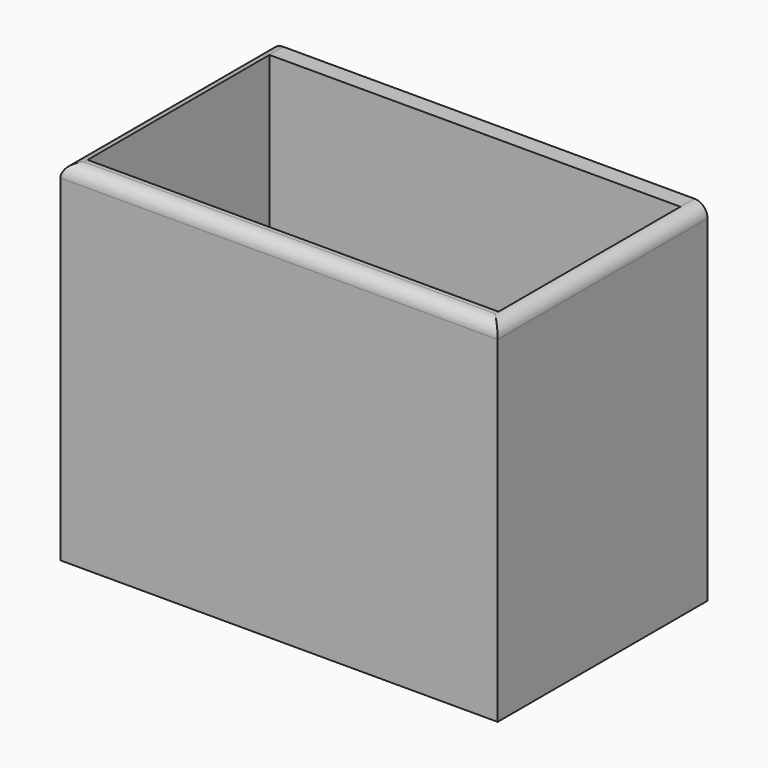
from build123d import *

# Parameters (mm, degrees)
F0_W     = 127
F0_H     = 76.2
F0_W_2   = 119.38
F0_H_2   = 66.04
F1_DEPTH = 101.6
F2_W     = 12.954
F2_H     = 17.78
F3_DEPTH = 5.08
F4_W     = 119.38
F4_H     = 66.04
F5_DEPTH = 3.81
F6_R     = 3.80999


# Not quite as in the source:
# - a fillet or chamfer is up to 0.001 mm smaller than in the source, because OpenCascade refuses the exact size


with BuildPart() as f1:
    # F0 (on Top) → F1 (new body)
    with BuildSketch(Plane.XY):
        Rectangle(F0_W, F0_H)
        Rectangle(F0_W_2, F0_H_2, mode=Mode.SUBTRACT)
    extrude(amount=F1_DEPTH)

    # F2 (on face) → F3 (cut, through all)
    with BuildSketch(Plane(origin=(0, 38.1, 0), x_dir=(-1, 0, 0), z_dir=(0, 1, 0))):
        with Locations((-37.973, 45.72)):
            Rectangle(F2_W, F2_H)
        with Locations((37.973, 45.72)):
            Rectangle(F2_W, F2_H)
    extrude(amount=-F3_DEPTH, mode=Mode.SUBTRACT)

    # F6 (radius 3.81 in the source; OpenCascade refuses exactly that, so slightly less here)
    f6_edges = [f1.edges().sort_by_distance(p)[0] for p in [
        (63.5, 0, 101.6),
        (0, -38.1, 101.6),
        (-63.5, 0, 101.6),
    ]]
    fillet(f6_edges, radius=F6_R)


with BuildPart() as f5:
    # F4 (on face) → F5 (new body)
    with BuildSketch(Plane(origin=(0, 0, 0), x_dir=(1, 0, 0), z_dir=(0, 0, -1))):
        Rectangle(F4_W, F4_H)
    extrude(amount=-F5_DEPTH)


solid = Compound([f1.part, f5.part])
